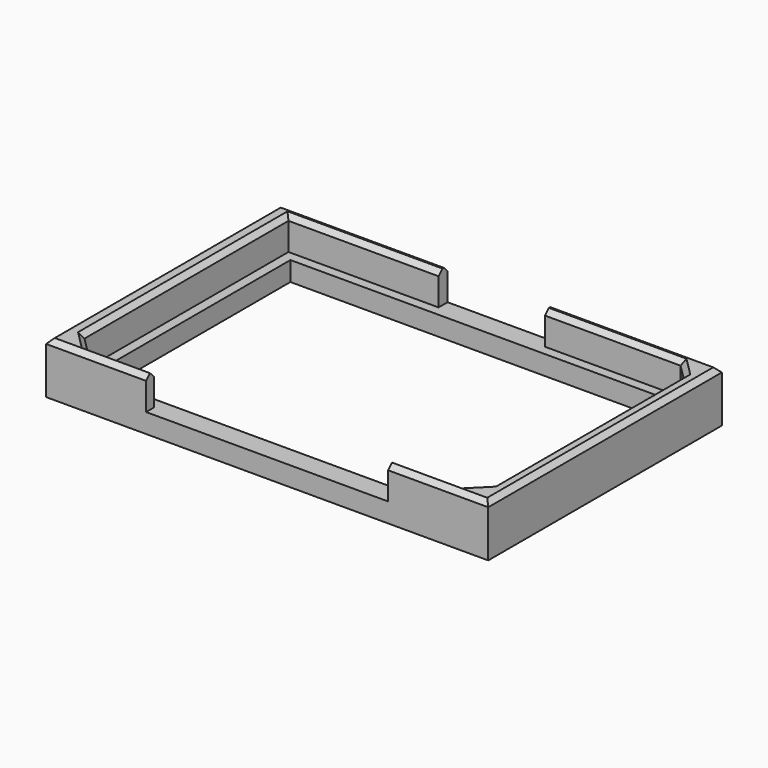
from build123d import *

# Parameters (mm, degrees)
F0_W     = 137
F0_H     = 90.5
F0_W_2   = 120.5
F0_H_2   = 77.5
F1_DEPTH = 16
F3_W     = 33
F3_H     = 20.2931881964
F3_H_2   = 28.397909285
F3_W_2   = 75
F3_H_3   = 9.5986060599
F3_H_4   = 10.4013939401
F4_DEPTH = 10
F5_SIZE  = 1.49999


# Not quite as in the source:
# - a fillet or chamfer is up to 0.001 mm smaller than in the source, because OpenCascade refuses the exact size
# - a feature names something its author has since deleted; it is built from what else it names


with BuildPart() as f1:
    # F0 (on Top) → F1 (new body)
    with BuildSketch(Plane.XY):
        with Locations((10.3103105978, 18.8386597227)):
            Rectangle(F0_W, F0_H)
        with Locations((10.5603105978, 18.8386597227)):
            Rectangle(F0_W_2, F0_H_2, mode=Mode.SUBTRACT)
    extrude(amount=F1_DEPTH)

    # F3 (on 3pt) → F4 (cut)
    with BuildSketch(Plane.XY.offset(16)):
        with Locations((10.3103105978, 70.7352538208)):
            Rectangle(F3_W, F3_H)
        with Locations((10.3103105978, 46.3897050802)):
            Rectangle(F3_W, F3_H_2)
        Polygon((-6.1896894022, 32.1907504376), (-6.1896894022, 60.5886597227), (-52.6896894022, 60.5886597227), (-52.6896894022, -18.4113402773), (-47.6896894022, -23.4113402773), (-27.1896894022, -23.4113402773), (-27.1896894022, -13.8127342174), (47.8103105978, -13.8127342174), (47.8103105978, -23.4113402773), (68.8103105978, -23.4113402773), (73.8103105978, -18.4113402773), (73.8103105978, 55.5886597227), (68.8103105978, 60.5886597227), (26.8103105978, 60.5886597227), (26.8103105978, 32.1907504376), align=None)
        with Locations((10.3103105978, -18.6120372474)):
            Rectangle(F3_W_2, F3_H_3)
        with Locations((10.3103105978, -28.6120372474)):
            Rectangle(F3_W_2, F3_H_4)
    extrude(amount=-F4_DEPTH, mode=Mode.SUBTRACT)

    # F5 (size 1.5 in the source; OpenCascade refuses exactly that, so slightly less here)
    f5_edges = [f1.edges().sort_by_distance(p)[0] for p in [
        (-52.689689, 21.08866, 16),
        (-29.439689, 60.58866, 16),
        (78.810311, 18.83866, 16),
        (63.310311, -26.41134, 16),
        (52.810311, 64.08866, 16),
        (-32.189689, 64.08866, 16),
        (-58.189689, 18.83866, 16),
        (-42.689689, -26.41134, 16),
        (71.310311, 58.08866, 16),
        (73.810311, 18.58866, 16),
        (71.310311, -20.91134, 16),
        (-50.189689, -20.91134, 16),
        (58.310311, -23.41134, 16),
        (47.810311, 60.58866, 16),
        (-37.439689, -23.41134, 16),
    ]]
    chamfer(f5_edges, length=F5_SIZE)


solid = f1.part
